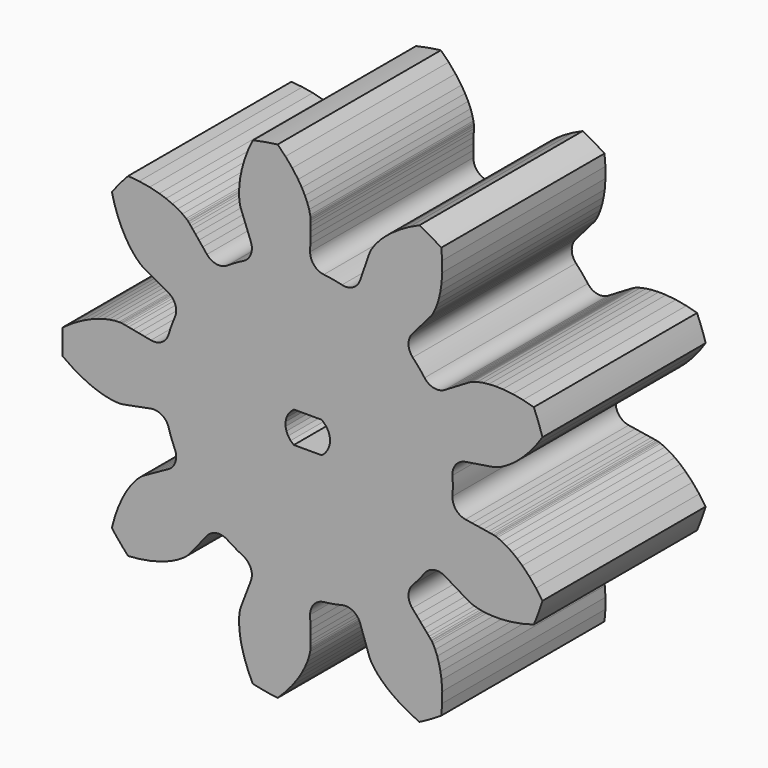
from build123d import *

# Parameters (mm, degrees)
F1_DEPTH = 18


# Not quite as in the source:
# - ends of sketch curves that miss each other by under 0.0002 mm in the source are joined


with BuildPart() as f1:
    # F0 (on Front) → F1 (new body)
    with BuildSketch(Plane.XZ):
        with BuildLine():
            Line((19.467552, -8.692774), (20.416309, -8.441776))
            ThreePointArc((20.416309, -8.441776), (20.8237645906, -7.4059478264), (21.1774532007, -6.3505500616))
            Line((21.1774532007, -6.3505500616), (20.612001, -5.548425))
            Line((20.612001, -5.548425), (20.017157, -4.830537))
            Line((20.017157, -4.830537), (19.404201, -4.200946))
            Line((19.404201, -4.200946), (18.931767, -3.783555))
            Line((18.931767, -3.783555), (18.463433, -3.424335))
            Line((18.463433, -3.424335), (18.008605, -3.126509))
            Line((18.008605, -3.126509), (17.580505, -2.89379))
            Line((17.580505, -2.89379), (17.20114, -2.73116))
            Line((17.20114, -2.73116), (17.074423, -2.688443))
            Line((17.074423, -2.688443), (16.976686, -2.660071))
            Line((16.976686, -2.660071), (16.925123, -2.64871))
            Line((16.925123, -2.64871), (16.806879, -2.627493))
            Line((16.806879, -2.627493), (16.618914, -2.595678))
            Line((16.618914, -2.595678), (16.368395, -2.554356))
            Line((16.368395, -2.554356), (15.970398, -2.489732))
            Line((15.970398, -2.489732), (15.49747, -2.413719))
            Line((15.49747, -2.413719), (14.964395, -2.328563))
            Line((14.964395, -2.328563), (14.385954, -2.236513))
            ThreePointArc((14.385954, -2.236513), (13.540102915, -1.7445781537), (13.2456102872, -0.8114450818))
            ThreePointArc((13.2456102872, -0.8114450818), (13.271366, 4.99e-07), (13.2456100847, 0.8114460689))
            ThreePointArc((13.2456100847, 0.8114460689), (13.540102866, 1.7445790924), (14.3859540035, 2.236512978))
            Line((14.3859540035, 2.236512978), (14.964395, 2.328564))
            Line((14.964395, 2.328564), (15.49747, 2.413719))
            Line((15.49747, 2.413719), (15.970398, 2.489732))
            Line((15.970398, 2.489732), (16.368395, 2.554356))
            Line((16.368395, 2.554356), (16.618914, 2.595679))
            Line((16.618914, 2.595679), (16.806879, 2.627494))
            Line((16.806879, 2.627494), (16.925123, 2.648711))
            Line((16.925123, 2.648711), (16.976686, 2.660072))
            Line((16.976686, 2.660072), (17.074423, 2.688444))
            Line((17.074423, 2.688444), (17.20114, 2.73116))
            Line((17.20114, 2.73116), (17.580505, 2.893791))
            Line((17.580505, 2.893791), (18.008605, 3.12651))
            Line((18.008605, 3.12651), (18.463433, 3.424336))
            Line((18.463433, 3.424336), (18.931767, 3.783556))
            Line((18.931767, 3.783556), (19.404201, 4.200947))
            Line((19.404201, 4.200947), (20.017157, 4.830538))
            Line((20.017157, 4.830538), (20.612001, 5.548425))
            Line((20.612001, 5.548425), (21.177453, 6.350551))
            ThreePointArc((21.177453, 6.350551), (20.8237644271, 7.4059482756), (20.4163091839, 8.4417760779))
            Line((20.4163091839, 8.4417760779), (19.467552, 8.692775))
            Line((19.467552, 8.692775), (18.550425, 8.86035))
            Line((18.550425, 8.86035), (17.676181, 8.948644))
            Line((17.676181, 8.948644), (17.045981, 8.964709))
            Line((17.045981, 8.964709), (16.456315, 8.938848))
            Line((16.456315, 8.938848), (15.916457, 8.874638))
            Line((15.916457, 8.874638), (15.438924, 8.777734))
            Line((15.438924, 8.777734), (15.043778, 8.658466))
            Line((15.043778, 8.658466), (14.919249, 8.609736))
            Line((14.919249, 8.609736), (14.826141, 8.568646))
            Line((14.826141, 8.568646), (14.779338, 8.544205))
            Line((14.779338, 8.544205), (14.675121, 8.484453))
            Line((14.675121, 8.484453), (14.51068, 8.388002))
            Line((14.51068, 8.388002), (14.29221, 8.258627))
            Line((14.29221, 8.258627), (13.945787, 8.052304))
            Line((13.945787, 8.052304), (13.534644, 7.806542))
            Line((13.534644, 7.806542), (13.071548, 7.52912))
            Line((13.071548, 7.52912), (12.569267, 7.227821))
            ThreePointArc((12.569267, 7.227821), (11.6050980187, 7.0609608944), (10.7796968527, 7.5864866278))
            ThreePointArc((10.7796968527, 7.5864866278), (10.2778396122, 8.2246454305), (9.7365222437, 8.8296932323))
            ThreePointArc((9.7365222437, 8.8296932323), (9.3623109596, 9.7338107708), (9.6940618683, 10.654356246))
            Line((9.6940618683, 10.654356246), (10.078004, 11.096687))
            Line((10.078004, 11.096687), (10.431626, 11.504574))
            Line((10.431626, 11.504574), (10.745049, 11.866795))
            Line((10.745049, 11.866795), (11.008394, 12.172128))
            Line((11.008394, 12.172128), (11.17374, 12.364813))
            Line((11.17374, 12.364813), (11.29728, 12.510006))
            Line((11.29728, 12.510006), (11.374222, 12.602265))
            Line((11.374222, 12.602265), (11.406419, 12.644112))
            Line((11.406419, 12.644112), (11.463052, 12.72867))
            Line((11.463052, 12.72867), (11.532666, 12.842846))
            Line((11.532666, 12.842846), (11.718739, 13.211278))
            Line((11.718739, 13.211278), (11.897094, 13.664729))
            Line((11.897094, 13.664729), (12.054073, 14.185235))
            Line((12.054073, 14.185235), (12.181936, 14.761452))
            Line((12.181936, 14.761452), (12.275548, 15.384868))
            Line((12.275548, 15.384868), (12.340406, 16.261163))
            Line((12.340406, 16.261163), (12.334634, 17.193455))
            Line((12.334634, 17.193455), (12.252199, 18.171384))
            ThreePointArc((12.252199, 18.171384), (11.3028611549, 18.7525185192), (10.3249147965, 19.2841016016))
            Line((10.3249147965, 19.2841016016), (9.436786, 18.866528))
            Line((9.436786, 18.866528), (8.626511, 18.405381))
            Line((8.626511, 18.405381), (7.900047, 17.911065))
            Line((7.900047, 17.911065), (7.406959, 17.518287))
            Line((7.406959, 17.518287), (6.971872, 17.119446))
            Line((6.971872, 17.119446), (6.59959, 16.723244))
            Line((6.59959, 16.723244), (6.296068, 16.342059))
            Line((6.296068, 16.342059), (6.070032, 15.996699))
            Line((6.070032, 15.996699), (6.00596, 15.879324))
            Line((6.00596, 15.879324), (5.961048, 15.787999))
            Line((5.961048, 15.787999), (5.940905, 15.739192))
            Line((5.940905, 15.739192), (5.899477, 15.626429))
            Line((5.899477, 15.626429), (5.835506, 15.446843))
            Line((5.835506, 15.446843), (5.751309, 15.207307))
            Line((5.751309, 15.207307), (5.618556, 14.826577))
            Line((5.618556, 14.826577), (5.461574, 14.374035))
            Line((5.461574, 14.374035), (5.285145, 13.863845))
            Line((5.285145, 13.863845), (5.094048, 13.310176))
            ThreePointArc((5.094048, 13.310176), (4.462706417, 12.5625981273), (3.4926110756, 12.4346163116))
            ThreePointArc((3.4926110756, 12.4346163116), (2.697966047, 12.600887062), (1.8943760505, 12.7164284528))
            ThreePointArc((1.8943760505, 12.7164284528), (1.0265568274, 13.1684839504), (0.6889772591, 14.0869089956))
            Line((0.6889772591, 14.0869089956), (0.69877, 14.672547))
            Line((0.69877, 14.672547), (0.707476, 15.21231))
            Line((0.707476, 15.21231), (0.714741, 15.691252))
            Line((0.714741, 15.691252), (0.72021, 16.094425))
            Line((0.72021, 16.094425), (0.723017, 16.348313))
            Line((0.723017, 16.348313), (0.724326, 16.538948))
            Line((0.724326, 16.538948), (0.723964, 16.659079))
            Line((0.723964, 16.659079), (0.721729, 16.711832))
            Line((0.721729, 16.711832), (0.71076, 16.81301))
            Line((0.71076, 16.81301), (0.690697, 16.945221))
            Line((0.690697, 16.945221), (0.596413, 17.347062))
            Line((0.596413, 17.347062), (0.441568, 17.80907))
            Line((0.441568, 17.80907), (0.227247, 18.308705))
            Line((0.227247, 18.308705), (-0.04519, 18.832302))
            Line((-0.04519, 18.832302), (-0.374203, 19.370038))
            Line((-0.374203, 19.370038), (-0.887791, 20.083009))
            Line((-0.887791, 20.083009), (-1.491478, 20.793476))
            Line((-1.491478, 20.793476), (-2.183227, 21.489625))
            ThreePointArc((-2.183227, 21.489625), (-3.2840082545, 21.3245770314), (-4.3748538771, 21.1031814652))
            Line((-4.3748538771, 21.1031814652), (-4.786789, 20.212424))
            Line((-4.786789, 20.212424), (-5.111075, 19.33833))
            Line((-5.111075, 19.33833), (-5.34984, 18.492699))
            Line((-5.34984, 18.492699), (-5.475094, 17.874863))
            Line((-5.475094, 17.874863), (-5.55202, 17.289664))
            Line((-5.55202, 17.289664), (-5.582531, 16.746858))
            Line((-5.582531, 16.746858), (-5.570022, 16.259753))
            Line((-5.570022, 16.259753), (-5.521182, 15.849899))
            Line((-5.521182, 15.849899), (-5.494816, 15.7188))
            Line((-5.494816, 15.7188), (-5.470519, 15.619972))
            Line((-5.470519, 15.619972), (-5.454576, 15.569636))
            Line((-5.454576, 15.569636), (-5.413829, 15.456626))
            Line((-5.413829, 15.456626), (-5.347399, 15.277935))
            Line((-5.347399, 15.277935), (-5.257926, 15.040319))
            Line((-5.257926, 15.040319), (-5.114893, 14.66333))
            Line((-5.114893, 14.66333), (-4.944259, 14.215757))
            Line((-4.944259, 14.215757), (-4.751468, 13.711523))
            Line((-4.751468, 13.711523), (-4.541965, 13.164553))
            ThreePointArc((-4.541965, 13.164553), (-4.5450671963, 12.1860563899), (-5.2059381265, 11.4644512552))
            ThreePointArc((-5.2059381265, 11.4644512552), (-5.9215480921, 11.0810340113), (-6.6114021781, 10.6530062678))
            ThreePointArc((-6.6114021781, 10.6530062678), (-7.5667658643, 10.4414778458), (-8.4157188515, 10.9280401204))
            Line((-8.4157188515, 10.9280401204), (-8.784658, 11.382959))
            Line((-8.784658, 11.382959), (-9.124943, 11.802038))
            Line((-9.124943, 11.802038), (-9.427235, 12.173598))
            Line((-9.427235, 12.173598), (-9.6822, 12.485963))
            Line((-9.6822, 12.485963), (-9.843246, 12.682257))
            Line((-9.843246, 12.682257), (-9.964781, 12.829132))
            Line((-9.964781, 12.829132), (-10.042277, 12.920925))
            Line((-10.042277, 12.920925), (-10.077898, 12.9599))
            Line((-10.077898, 12.9599), (-10.151337, 13.030357))
            Line((-10.151337, 13.030357), (-10.251689, 13.118739))
            Line((-10.251689, 13.118739), (-10.582214, 13.365963))
            Line((-10.582214, 13.365963), (-10.997804, 13.620349))
            Line((-10.997804, 13.620349), (-11.483144, 13.865329))
            Line((-11.483144, 13.865329), (-12.028404, 14.091308))
            Line((-12.028404, 14.091308), (-12.626092, 14.291752))
            Line((-12.626092, 14.291752), (-13.477812, 14.507792))
            Line((-13.477812, 14.507792), (-14.396943, 14.663999))
            Line((-14.396943, 14.663999), (-15.37433, 14.752632))
            ThreePointArc((-15.37433, 14.752632), (-16.1114862641, 13.9186291759), (-16.8048121234, 13.0478483381))
            Line((-16.8048121234, 13.0478483381), (-16.547805, 12.100702))
            Line((-16.547805, 12.100702), (-16.234366, 11.22266))
            Line((-16.234366, 11.22266), (-15.873709, 10.421394))
            Line((-15.873709, 10.421394), (-15.572521, 9.867593))
            Line((-15.572521, 9.867593), (-15.255292, 9.369857))
            Line((-15.255292, 9.369857), (-14.929756, 8.934431))
            Line((-14.929756, 8.934431), (-14.607068, 8.569328))
            Line((-14.607068, 8.569328), (-14.306205, 8.286755))
            Line((-14.306205, 8.286755), (-14.201739, 8.203275))
            Line((-14.201739, 8.203275), (-14.1196, 8.143186))
            Line((-14.1196, 8.143186), (-14.075033, 8.114875))
            Line((-14.075033, 8.114875), (-13.971177, 8.054495))
            Line((-13.971177, 8.054495), (-13.805428, 7.960311))
            Line((-13.805428, 7.960311), (-13.584151, 7.835798))
            Line((-13.584151, 7.835798), (-13.232258, 7.638949))
            Line((-13.232258, 7.638949), (-12.81385, 7.405769))
            Line((-12.81385, 7.405769), (-12.342048, 7.143427))
            Line((-12.342048, 7.143427), (-11.829975, 6.859089))
            ThreePointArc((-11.829975, 6.859089), (-11.2033854167, 6.1075239385), (-11.2458025612, 5.129942808))
            ThreePointArc((-11.2458025612, 5.129942808), (-11.5475362774, 4.3762425729), (-11.8008644256, 3.604924125))
            ThreePointArc((-11.8008644256, 3.604924125), (-12.3967476489, 2.828787613), (-13.3598400496, 2.655819744))
            Line((-13.3598400496, 2.655819744), (-13.93488, 2.767159))
            Line((-13.93488, 2.767159), (-14.464931, 2.869461))
            Line((-14.464931, 2.869461), (-14.935335, 2.959783))
            Line((-14.935335, 2.959783), (-15.331434, 3.035179))
            Line((-15.331434, 3.035179), (-15.580977, 3.082031))
            Line((-15.580977, 3.082031), (-15.768488, 3.116423))
            Line((-15.768488, 3.116423), (-15.886857, 3.136927))
            Line((-15.886857, 3.136927), (-15.939197, 3.143887))
            Line((-15.939197, 3.143887), (-16.040743, 3.150654))
            Line((-16.040743, 3.150654), (-16.174429, 3.153854))
            Line((-16.174429, 3.153854), (-16.586537, 3.130781))
            Line((-16.586537, 3.130781), (-17.068414, 3.058516))
            Line((-17.068414, 3.058516), (-17.597676, 2.934211))
            Line((-17.597676, 2.934211), (-18.160626, 2.756834))
            Line((-18.160626, 2.756834), (-18.747325, 2.526197))
            Line((-18.747325, 2.526197), (-19.538648, 2.144218))
            Line((-19.538648, 2.144218), (-20.343151, 1.673074))
            Line((-20.343151, 1.673074), (-21.148845, 1.112718))
            ThreePointArc((-21.148845, 1.112718), (-21.177453, 0), (-21.1488442932, -1.1127179636))
            Line((-21.1488442932, -1.1127179636), (-20.343151, -1.673073))
            Line((-20.343151, -1.673073), (-19.538648, -2.144218))
            Line((-19.538648, -2.144218), (-18.747325, -2.526197))
            Line((-18.747325, -2.526197), (-18.160626, -2.756834))
            Line((-18.160626, -2.756834), (-17.597676, -2.93421))
            Line((-17.597676, -2.93421), (-17.068414, -3.058515))
            Line((-17.068414, -3.058515), (-16.586537, -3.13078))
            Line((-16.586537, -3.13078), (-16.174429, -3.153853))
            Line((-16.174429, -3.153853), (-16.040743, -3.150654))
            Line((-16.040743, -3.150654), (-15.939197, -3.143886))
            Line((-15.939197, -3.143886), (-15.886857, -3.136927))
            Line((-15.886857, -3.136927), (-15.768488, -3.116423))
            Line((-15.768488, -3.116423), (-15.580977, -3.082031))
            Line((-15.580977, -3.082031), (-15.331434, -3.035179))
            Line((-15.331434, -3.035179), (-14.935335, -2.959782))
            Line((-14.935335, -2.959782), (-14.464931, -2.86946))
            Line((-14.464931, -2.86946), (-13.93488, -2.767158))
            Line((-13.93488, -2.767158), (-13.35984, -2.655819))
            ThreePointArc((-13.35984, -2.655819), (-12.3967479774, -2.828787413), (-11.8008644856, -3.6049231426))
            ThreePointArc((-11.8008644856, -3.6049231426), (-11.5475365982, -4.3762416917), (-11.2458032681, -5.1299421173))
            ThreePointArc((-11.2458032681, -5.1299421173), (-11.2033851924, -6.1075232747), (-11.8299748964, -6.8590881866))
            Line((-11.8299748964, -6.8590881866), (-12.342048, -7.143426))
            Line((-12.342048, -7.143426), (-12.81385, -7.405768))
            Line((-12.81385, -7.405768), (-13.232258, -7.638948))
            Line((-13.232258, -7.638948), (-13.584151, -7.835798))
            Line((-13.584151, -7.835798), (-13.805428, -7.960311))
            Line((-13.805428, -7.960311), (-13.971177, -8.054495))
            Line((-13.971177, -8.054495), (-14.075033, -8.114874))
            Line((-14.075033, -8.114874), (-14.1196, -8.143186))
            Line((-14.1196, -8.143186), (-14.201739, -8.203274))
            Line((-14.201739, -8.203274), (-14.306205, -8.286755))
            Line((-14.306205, -8.286755), (-14.607068, -8.569328))
            Line((-14.607068, -8.569328), (-14.929756, -8.934431))
            Line((-14.929756, -8.934431), (-15.255292, -9.369856))
            Line((-15.255292, -9.369856), (-15.572521, -9.867592))
            Line((-15.572521, -9.867592), (-15.873709, -10.421394))
            Line((-15.873709, -10.421394), (-16.234366, -11.222659))
            Line((-16.234366, -11.222659), (-16.547805, -12.100701))
            Line((-16.547805, -12.100701), (-16.804813, -13.047848))
            ThreePointArc((-16.804813, -13.047848), (-16.1114867558, -13.9186285898), (-15.3743298116, -14.7526308247))
            Line((-15.3743298116, -14.7526308247), (-14.396943, -14.663998))
            Line((-14.396943, -14.663998), (-13.477812, -14.507791))
            Line((-13.477812, -14.507791), (-12.626092, -14.291752))
            Line((-12.626092, -14.291752), (-12.028404, -14.091307))
            Line((-12.028404, -14.091307), (-11.483144, -13.865328))
            Line((-11.483144, -13.865328), (-10.997804, -13.620348))
            Line((-10.997804, -13.620348), (-10.582214, -13.365962))
            Line((-10.582214, -13.365962), (-10.251689, -13.118738))
            Line((-10.251689, -13.118738), (-10.151337, -13.030356))
            Line((-10.151337, -13.030356), (-10.077898, -12.959899))
            Line((-10.077898, -12.959899), (-10.042277, -12.920925))
            Line((-10.042277, -12.920925), (-9.964781, -12.829132))
            Line((-9.964781, -12.829132), (-9.843246, -12.682256))
            Line((-9.843246, -12.682256), (-9.6822, -12.485962))
            Line((-9.6822, -12.485962), (-9.427235, -12.173598))
            Line((-9.427235, -12.173598), (-9.124943, -11.802037))
            Line((-9.124943, -11.802037), (-8.784658, -11.382959))
            Line((-8.784658, -11.382959), (-8.415719, -10.928039))
            ThreePointArc((-8.415719, -10.928039), (-7.5667658643, -10.4414768458), (-6.6114021975, -10.6530052968))
            ThreePointArc((-6.6114021975, -10.6530052968), (-5.9215483319, -11.0810338728), (-5.205938156, -11.4644513148))
            ThreePointArc((-5.205938156, -11.4644513148), (-4.5450673662, -12.186055955), (-4.5419658331, -13.1645516807))
            Line((-4.5419658331, -13.1645516807), (-4.751468, -13.711522))
            Line((-4.751468, -13.711522), (-4.944259, -14.215756))
            Line((-4.944259, -14.215756), (-5.114893, -14.66333))
            Line((-5.114893, -14.66333), (-5.257926, -15.040318))
            Line((-5.257926, -15.040318), (-5.347399, -15.277935))
            Line((-5.347399, -15.277935), (-5.413829, -15.456625))
            Line((-5.413829, -15.456625), (-5.454576, -15.569635))
            Line((-5.454576, -15.569635), (-5.470519, -15.619971))
            Line((-5.470519, -15.619971), (-5.494816, -15.718799))
            Line((-5.494816, -15.718799), (-5.521182, -15.849898))
            Line((-5.521182, -15.849898), (-5.570022, -16.259753))
            Line((-5.570022, -16.259753), (-5.582531, -16.746858))
            Line((-5.582531, -16.746858), (-5.55202, -17.289664))
            Line((-5.55202, -17.289664), (-5.475094, -17.874863))
            Line((-5.475094, -17.874863), (-5.34984, -18.492698))
            Line((-5.34984, -18.492698), (-5.111075, -19.338329))
            Line((-5.111075, -19.338329), (-4.786789, -20.212423))
            Line((-4.786789, -20.212423), (-4.374854, -21.103181))
            ThreePointArc((-4.374854, -21.103181), (-3.2840084253, -21.3245770013), (-2.1832270507, -21.4896244099))
            Line((-2.1832270507, -21.4896244099), (-1.491478, -20.793476))
            Line((-1.491478, -20.793476), (-0.887791, -20.083008))
            Line((-0.887791, -20.083008), (-0.374203, -19.370037))
            Line((-0.374203, -19.370037), (-0.04519, -18.832301))
            Line((-0.04519, -18.832301), (0.227247, -18.308704))
            Line((0.227247, -18.308704), (0.441568, -17.809069))
            Line((0.441568, -17.809069), (0.596413, -17.347061))
            Line((0.596413, -17.347061), (0.690697, -16.94522))
            Line((0.690697, -16.94522), (0.71076, -16.81301))
            Line((0.71076, -16.81301), (0.721729, -16.711831))
            Line((0.721729, -16.711831), (0.723964, -16.659079))
            Line((0.723964, -16.659079), (0.724326, -16.538947))
            Line((0.724326, -16.538947), (0.723017, -16.348313))
            Line((0.723017, -16.348313), (0.72021, -16.094425))
            Line((0.72021, -16.094425), (0.714741, -15.691252))
            Line((0.714741, -15.691252), (0.707476, -15.21231))
            Line((0.707476, -15.21231), (0.69877, -14.672546))
            Line((0.69877, -14.672546), (0.688977, -14.086908))
            ThreePointArc((0.688977, -14.086908), (1.0265571576, -13.168483575), (1.8943760267, -12.7164282393))
            ThreePointArc((1.8943760267, -12.7164282393), (2.697966047, -12.600887062), (3.4926111281, -12.4346165281))
            ThreePointArc((3.4926111281, -12.4346165281), (4.462706417, -12.5625981273), (5.0940472591, -13.3101762555))
            Line((5.0940472591, -13.3101762555), (5.285145, -13.863845))
            Line((5.285145, -13.863845), (5.461574, -14.374034))
            Line((5.461574, -14.374034), (5.618556, -14.826577))
            Line((5.618556, -14.826577), (5.751309, -15.207306))
            Line((5.751309, -15.207306), (5.835506, -15.446843))
            Line((5.835506, -15.446843), (5.899477, -15.626428))
            Line((5.899477, -15.626428), (5.940905, -15.739191))
            Line((5.940905, -15.739191), (5.961048, -15.787998))
            Line((5.961048, -15.787998), (6.00596, -15.879323))
            Line((6.00596, -15.879323), (6.070032, -15.996698))
            Line((6.070032, -15.996698), (6.296068, -16.342059))
            Line((6.296068, -16.342059), (6.59959, -16.723244))
            Line((6.59959, -16.723244), (6.971872, -17.119445))
            Line((6.971872, -17.119445), (7.406959, -17.518286))
            Line((7.406959, -17.518286), (7.900047, -17.911064))
            Line((7.900047, -17.911064), (8.626511, -18.40538))
            Line((8.626511, -18.40538), (9.436786, -18.866528))
            Line((9.436786, -18.866528), (10.324915, -19.284101))
            ThreePointArc((10.324915, -19.284101), (11.3028615874, -18.7525182695), (12.2521992655, -18.1713834096))
            Line((12.2521992655, -18.1713834096), (12.334634, -17.193454))
            Line((12.334634, -17.193454), (12.340406, -16.261162))
            Line((12.340406, -16.261162), (12.275548, -15.384867))
            Line((12.275548, -15.384867), (12.181936, -14.761452))
            Line((12.181936, -14.761452), (12.054073, -14.185234))
            Line((12.054073, -14.185234), (11.897094, -13.664728))
            Line((11.897094, -13.664728), (11.718739, -13.211278))
            Line((11.718739, -13.211278), (11.532666, -12.842845))
            Line((11.532666, -12.842845), (11.463052, -12.728669))
            Line((11.463052, -12.728669), (11.406419, -12.644112))
            Line((11.406419, -12.644112), (11.374222, -12.602264))
            Line((11.374222, -12.602264), (11.29728, -12.510006))
            Line((11.29728, -12.510006), (11.17374, -12.364812))
            Line((11.17374, -12.364812), (11.008394, -12.172127))
            Line((11.008394, -12.172127), (10.745049, -11.866794))
            Line((10.745049, -11.866794), (10.431626, -11.504573))
            Line((10.431626, -11.504573), (10.078004, -11.096686))
            Line((10.078004, -11.096686), (9.694061, -10.654356))
            ThreePointArc((9.694061, -10.654356), (9.3623109768, -9.7338100316), (9.7365227135, -8.8296926803))
            ThreePointArc((9.7365227135, -8.8296926803), (10.2778401036, -8.2246448448), (10.7796971535, -7.5864858493))
            ThreePointArc((10.7796971535, -7.5864858493), (11.6050981613, -7.0609608659), (12.5692667498, -7.2278204169))
            Line((12.5692667498, -7.2278204169), (13.071548, -7.52912))
            Line((13.071548, -7.52912), (13.534644, -7.806541))
            Line((13.534644, -7.806541), (13.945787, -8.052303))
            Line((13.945787, -8.052303), (14.29221, -8.258627))
            Line((14.29221, -8.258627), (14.51068, -8.388002))
            Line((14.51068, -8.388002), (14.675121, -8.484452))
            Line((14.675121, -8.484452), (14.779338, -8.544204))
            Line((14.779338, -8.544204), (14.826141, -8.568645))
            Line((14.826141, -8.568645), (14.919249, -8.609735))
            Line((14.919249, -8.609735), (15.043778, -8.658465))
            Line((15.043778, -8.658465), (15.438924, -8.777733))
            Line((15.438924, -8.777733), (15.916457, -8.874638))
            Line((15.916457, -8.874638), (16.456315, -8.938848))
            Line((16.456315, -8.938848), (17.045981, -8.964709))
            Line((17.045981, -8.964709), (17.676181, -8.948644))
            Line((17.676181, -8.948644), (18.550425, -8.860349))
            Line((18.550425, -8.860349), (19.467552, -8.692774))
        make_face()
        Polygon((1.984939, -1.13276), (1.704821, -1.377952), (-0.752641, -1.377952), (-1.03276, -1.13276), (-1.253165, -0.842738), (-1.405134, -0.519363), (-1.482652, -0.175435), (-1.482652, 0.175436), (-1.405134, 0.519364), (-1.253165, 0.842738), (-1.03276, 1.13276), (-0.752641, 1.377953), (1.704821, 1.377953), (1.984939, 1.13276), (2.205344, 0.842738), (2.357313, 0.519364), (2.434831, 0.175436), (2.434831, -0.175435), (2.357313, -0.519363), (2.205344, -0.842738), align=None, mode=Mode.SUBTRACT)
    extrude(amount=F1_DEPTH)


solid = f1.part
